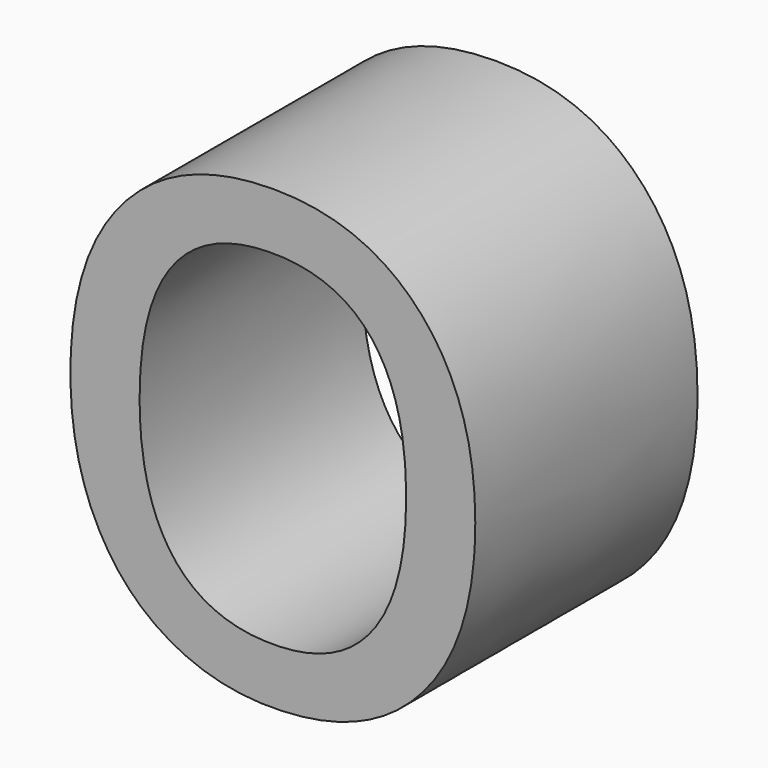
from build123d import *

# Parameters (mm, degrees)
F0_TEXT_SIZE = 37.6481019581
F1_DEPTH     = 12.7


# Not quite as in the source:
# - Text() gives the source's letters only with a copy of the font that has no kerning and outlines rounded to 1/6400 em; it was checked with that copy


with BuildPart() as f1:
    # F0 (on Front) → F1 (new body)
    with BuildSketch(Plane.XZ):
        with Locations((-54.6703968078, 0)):
            Text('o', F0_TEXT_SIZE, font='Open Sans', text_align=(TextAlign.LEFT, TextAlign.BOTTOM))
    extrude(amount=F1_DEPTH)


solid = f1.part
